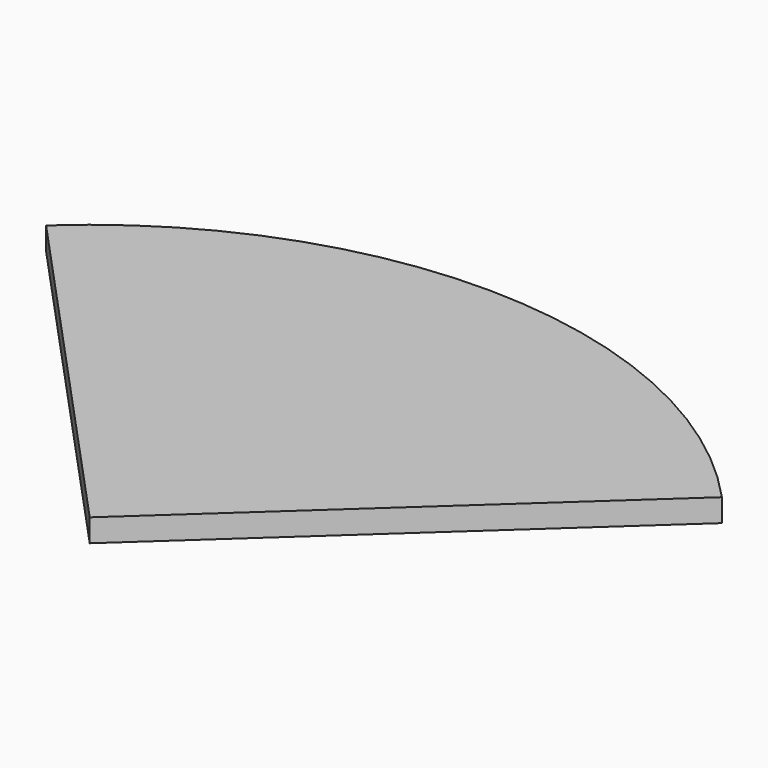
from build123d import *

# Parameters (mm, degrees)
F1_DEPTH = 18
F3_D     = 8
F3_DEPTH = 11
F3_TIP   = 2.4034424761


# Not quite as in the source:
# - a feature names something its author has since deleted; it is built from what else it names


with BuildPart() as f1:
    # F0 (on Top) → F1 (new body)
    with BuildSketch(Plane.XY):
        with BuildLine():
            ThreePointArc((287.0371856283, 264.0258587081), (16.2714653094, 389.6604155116), (-264.0258587081, 287.0371856283))
            Line((-264.0258587081, 287.0371856283), (0, 0))
            Line((0, 0), (287.0371856283, 264.0258587081))
        make_face()
    extrude(amount=F1_DEPTH)

    # F3
    with Locations(Plane(origin=(0, 0, 0), x_dir=(1, 0, 0), z_dir=(0, 0, -1))):
        with Locations((-111.8492066751, -134.8916415726), (-52.612635811, -70.4922730022), (58.3064641387, -65.860505917), (122.7058327092, -125.097076781), (187.1052012796, -184.333647645), (-171.0857775391, -199.2910101431)):
            Hole(F3_D / 2, depth=F3_DEPTH)
            with Locations((0, 0, -(F3_DEPTH + F3_TIP / 2))):  # 118° drill point
                Cone(0, F3_D / 2, F3_TIP, mode=Mode.SUBTRACT)


solid = f1.part
